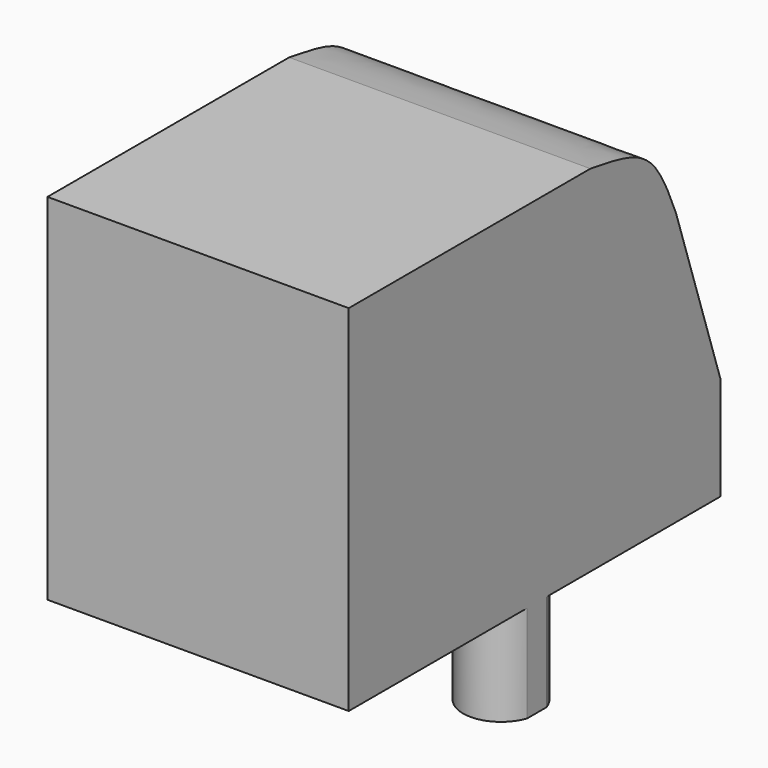
from build123d import *

# Parameters (mm, degrees)
F0_W     = 13.335
F0_H     = 15.7
F1_DEPTH = 20.57
F3_DEPTH = 4.3
F5_DEPTH = 13.336


with BuildPart() as f1:
    # F0 (on Front) → F1 (new body)
    with BuildSketch(Plane.XZ):
        Rectangle(F0_W, F0_H)
    extrude(amount=-F1_DEPTH)

    # F2 (on face) → F3 (join)
    with BuildSketch(Plane(origin=(0, 0, -7.85), x_dir=(1, 0, 0), z_dir=(0, 0, -1))):
        with BuildLine():
            Line((6.6675, -10.9442927568), (6.6675, -9.8757072432))
            ThreePointArc((6.6675, -9.8757072432), (3.405, -10.41), (6.6675, -10.9442927568))
        make_face()
        with BuildLine():
            ThreePointArc((-3.405, -10.41), (-4.8092949022, -8.757019737), (-6.6675, -9.8757072432))
            Line((-6.6675, -9.8757072432), (-6.6675, -10.9442927568))
            ThreePointArc((-6.6675, -10.9442927568), (-4.8092949022, -12.062980263), (-3.405, -10.41))
        make_face()
    extrude(amount=F3_DEPTH)

    # F4 (on face) → F5 (cut, through all)
    with BuildSketch(Plane.YZ.offset(6.6675)):
        with BuildLine():
            Line((18.1063264608, 4.1939658113), (20.57, -3.2797483727))
            Line((20.57, -3.2797483727), (20.57, 7.85))
            Line((20.57, 7.85), (13.3700780571, 7.85))
            add(Edge.make_bspline(
                [(18.1063264608, 4.1939658113), (16.9114023447, 7.1921413764), (16.3248032331, 7.3876748793), (13.3700780571, 7.85)],
                knots=[0, 0, 0, 0, 5.9831960466, 5.9831960466, 5.9831960466, 5.9831960466], degree=3))
        make_face()
    extrude(amount=-F5_DEPTH, mode=Mode.SUBTRACT)


solid = f1.part
